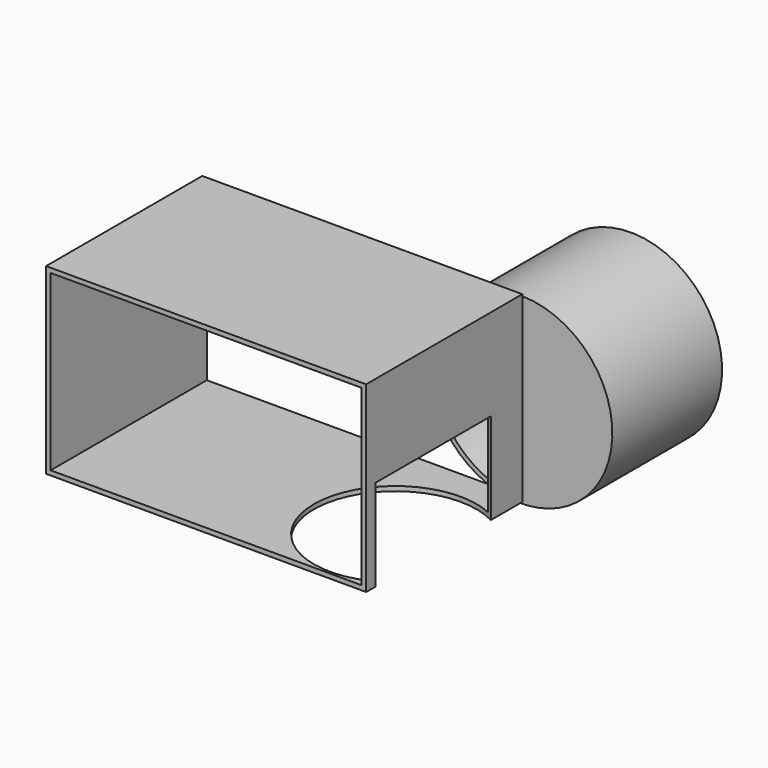
from build123d import *

# Parameters (mm, degrees)
F0_W        = 177.8
F0_H        = 108.4261015058
F1_DEPTH    = 101.6
F2_R        = 50.7821410518
F3_DEPTH    = 76.2
F6_T        = 2.54
F6_T3_DEPTH = 15.513104752
F6_T5_DEPTH = 105.7102081755
F7_R        = 45.225137574
F8_DEPTH    = 50.8


# Not quite as in the source:
# - a feature of the source that left no trace in its solid (it failed there, or was rolled back) is left out
# - a shell that OpenCascade refuses in one call is made with other operations: the cavity is built on its own and cut out


with BuildPart() as f1:
    # F0 (on Top) → F1 (new body)
    with BuildSketch(Plane.XY):
        with Locations((-74.0991531372, 54.2130507529)):
            Rectangle(F0_W, F0_H)
    extrude(amount=F1_DEPTH)

    # F2 (on face) → F3 (join)
    with BuildSketch(Plane(origin=(0, 108.4261015058, 0), x_dir=(-1, 0, 0), z_dir=(0, 1, 0))):
        with Locations((-14.0330018476, 49.8538725078)):
            Circle(F2_R)
    extrude(amount=F3_DEPTH)

    # F6: shell of thickness 2.54, made by hand


with BuildPart() as f6_core1:
    # F6_t2: copy of F1
    add(f1.part)

    # the walls: a layer under each face that stays
    f6_faces = [f6_core1.faces().sort_by_distance(p)[0] for p in [
        (64.8151428994, 146.5261015058, 49.8538725078),
        (-74.0991531372, 54.2130507529, 0),
        (-162.9991531372, 54.2130507529, 50.8),
        (-74.0991531372, 54.2130507529, 101.6),
        (14.8008468628, 54.2130507529, 50.8),
        (34.5914425051, 108.4261015058, 49.8509698158),
    ]]
    thicken(f6_faces, amount=-F6_T, mode=Mode.SUBTRACT)

    # F6_s4 → F6_t3 (cut)
    with BuildSketch(Plane.YZ.offset(1.8277421108)):
        Polygon((108.4007015058, -0.0254), (108.4261015058, 2.54), (110.9661015058, 2.54), (110.9661015058, 0), align=None)
    extrude(amount=F6_T3_DEPTH, mode=Mode.SUBTRACT)

    # F6_s6 → F6_t5 (cut)
    with BuildSketch(Plane.XY.offset(-2.54)):
        Polygon((14.8262468628, 108.4007015058), (12.2608468628, 108.4261015058), (12.2608468628, 110.9661015058), (14.8008468628, 110.9661015058), align=None)
    extrude(amount=F6_T5_DEPTH, mode=Mode.SUBTRACT)


with BuildPart() as f1_1:
    add(f1.part)

    # what is left inside the walls is the cavity
    f6_cavity = [f6_core1.part.solids().sort_by_distance(p)[0] for p in [
        (62.249743, 159.226102, 49.853873),
    ]]
    add(f6_cavity, mode=Mode.SUBTRACT)

    # F7 (on face) → F8 (cut)
    with BuildSketch(Plane(origin=(0, 0, 0), x_dir=(1, 0, 0), z_dir=(0, 0, -1))):
        with Locations((-6.2627755105, -46.561319381)):
            Circle(F7_R)
    extrude(amount=-F8_DEPTH, mode=Mode.SUBTRACT)


solid = f1_1.part
